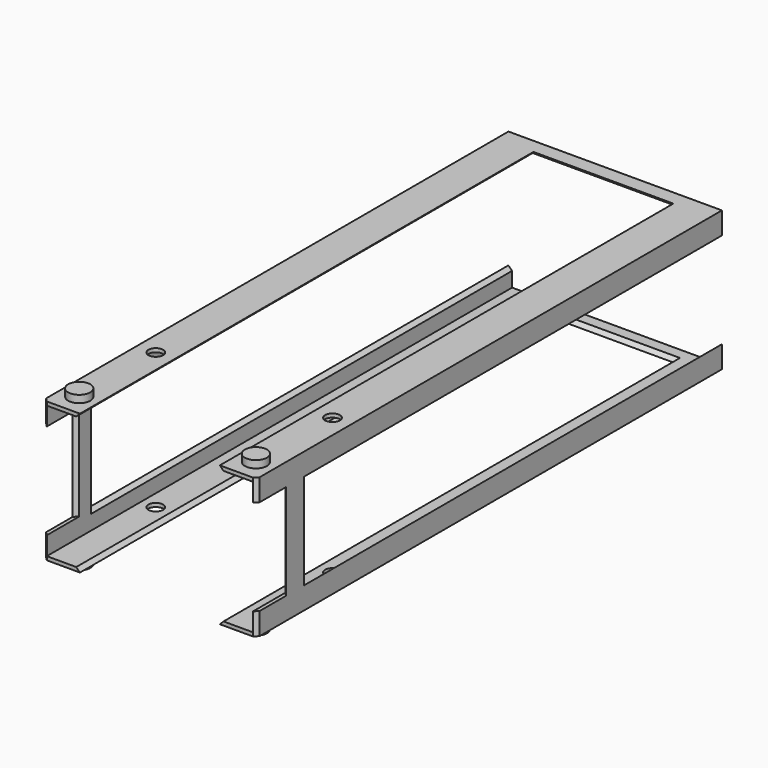
from build123d import *

# Parameters (mm, degrees)
F0_W     = 29
F0_H     = 79
F0_R     = 1.5
F0_R_2   = 1
F1_DEPTH = 9.5
F2_DEPTH = 10.5
F3_W     = 0.5
F3_H     = 13
F3_W_2   = 19
F3_H_2   = 0.5
F4_DEPTH = 77
F5_DEPTH = 79
F6_DEPTH = 8
F7_DEPTH = 5
F8_SIZE2 = 0.49999
F8_SIZE  = 0.49999


# Not quite as in the source:
# - a fillet or chamfer is up to 0.001 mm smaller than in the source, because OpenCascade refuses the exact size


with BuildPart() as f1:
    # F0 (on Top) → F1 (new body, symmetric)
    with BuildSketch(Plane.XY):
        with Locations((0, 39.5)):
            Rectangle(F0_W, F0_H)
        with Locations((-12, 3)):
            Circle(F0_R, mode=Mode.SUBTRACT)
        with Locations((-12, 16)):
            Circle(F0_R_2, mode=Mode.SUBTRACT)
        with Locations((12, 3)):
            Circle(F0_R, mode=Mode.SUBTRACT)
        with Locations((12, 16)):
            Circle(F0_R_2, mode=Mode.SUBTRACT)
    extrude(amount=F1_DEPTH, both=True)

    # F0 (on Top) → F2 (join, symmetric)
    with BuildSketch(Plane.XY):
        with Locations((-12, 3)):
            Circle(F0_R)
        with Locations((12, 3)):
            Circle(F0_R)
    extrude(amount=F2_DEPTH, both=True)

    # F3 (on Front) → F4 (cut)
    with BuildSketch(Plane.XZ):
        Polygon((9.5, 9), (-9.5, 9), (-14, 9), (-14, 6.5), (-14, -6.5), (-14, -9), (-9.5, -9), (9.5, -9), (14, -9), (14, -6.5), (14, 6.5), (14, 9), align=None)
        with Locations((-14.25, 0)):
            Rectangle(F3_W, F3_H)
        with Locations((0, 9.25)):
            Rectangle(F3_W_2, F3_H_2)
        with Locations((14.25, 0)):
            Rectangle(F3_W, F3_H)
        with Locations((0, -9.25)):
            Rectangle(F3_W_2, F3_H_2)
    extrude(amount=-F4_DEPTH, mode=Mode.SUBTRACT)

    # F3 (on Front) → F5 (cut)
    with BuildSketch(Plane.XZ):
        Polygon((9.5, 9), (-9.5, 9), (-14, 9), (-14, 6.5), (-14, -6.5), (-14, -9), (-9.5, -9), (9.5, -9), (14, -9), (14, -6.5), (14, 6.5), (14, 9), align=None)
        with Locations((-14.25, 0)):
            Rectangle(F3_W, F3_H)
        with Locations((14.25, 0)):
            Rectangle(F3_W, F3_H)
    extrude(amount=-F5_DEPTH, mode=Mode.SUBTRACT)

    # F3 (on Front) → F6 (join)
    with BuildSketch(Plane.XZ):
        with Locations((-14.25, 0)):
            Rectangle(F3_W, F3_H)
        with Locations((14.25, 0)):
            Rectangle(F3_W, F3_H)
    extrude(amount=-F6_DEPTH)

    # F3 (on Front) → F7 (cut)
    with BuildSketch(Plane.XZ):
        with Locations((-14.25, 0)):
            Rectangle(F3_W, F3_H)
        with Locations((14.25, 0)):
            Rectangle(F3_W, F3_H)
    extrude(amount=-F7_DEPTH, mode=Mode.SUBTRACT)

    # F8 (size 0.5 and 0.5 in the source; OpenCascade refuses exactly that, so slightly less here)
    f8_edges = [f1.edges().sort_by_distance(p)[0] for p in [
        (-9.5, 38.5, -9),
        (9.5, 38.5, -9),
        (14, 43.5, -6.5),
        (-14, 43.5, -6.5),
        (14, 43.5, 6.5),
        (9.5, 38.5, 9),
        (-14, 43.5, 6.5),
        (-9.5, 38.5, 9),
        (14.5, 0, -8),
        (14.5, 0, 8),
        (-14.5, 0, -8),
        (-14.5, 0, 8),
        (-14, 5, 0),
        (14, 5, 0),
        (-14, 8, 0),
        (14, 8, 0),
        (0, 77, -9),
        (0, 77, 9),
    ]]
    chamfer(f8_edges, length=F8_SIZE, length2=F8_SIZE2)


solid = f1.part
